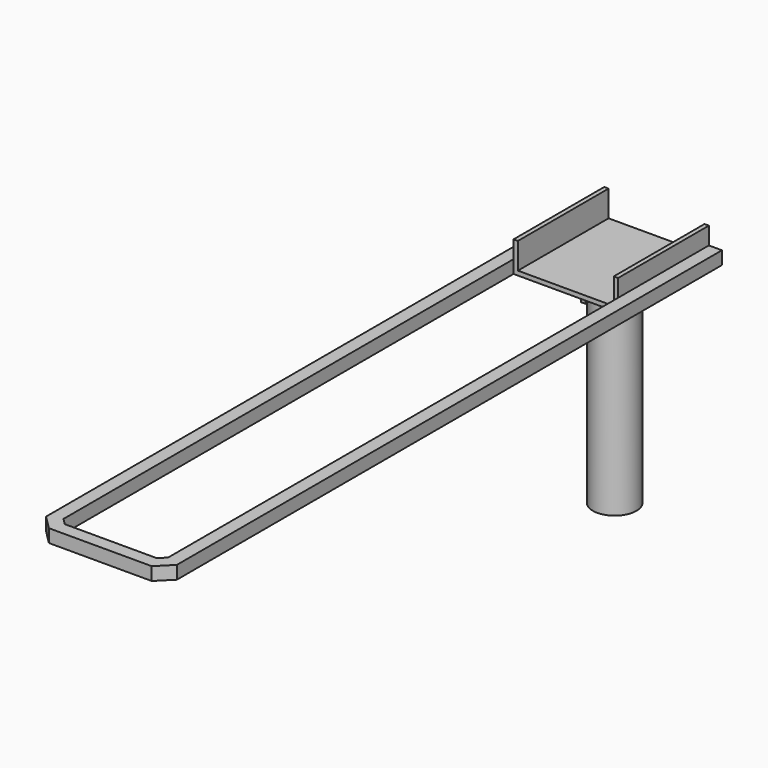
from build123d import *

# Parameters (mm, degrees)
F0_R     = 31.75
F0_R_2   = 28.575
F1_DEPTH = 304.8
F2_W     = 6.35
F2_H     = 28.575
F3_DEPTH = 25.4
F6_DEPTH = 165.1
F7_W     = 19.05
F7_H     = 19.05
F7_W_2   = 12.7
F7_H_2   = 12.7


# Not quite as in the source:
# - a feature names something its author has since deleted; it is built from what else it names


with BuildPart() as f1:
    # F0 (on Top) → F1 (new body)
    with BuildSketch(Plane.XY):
        Circle(F0_R)
        Circle(F0_R_2, mode=Mode.SUBTRACT)
    extrude(amount=-F1_DEPTH)

    # F2 (on Top) → F3 (join)
    with BuildSketch(Plane.XY):
        with Locations((0, -42.8625)):
            Rectangle(F2_W, F2_H)
    extrude(amount=-F3_DEPTH)

    # F5 (on offset) → F6 (join)
    with BuildSketch(Plane.XZ.offset(-76.2)):
        Polygon((-76.2, 0), (76.2, 0), (76.2, 44.45), (69.85, 44.45), (69.85, 6.35), (-69.85, 6.35), (-69.85, 44.45), (-76.2, 44.45), align=None)
    extrude(amount=F6_DEPTH)

    # F9: sweep along a path in F8
    with BuildLine(Plane.XY.offset(6.35)) as f9_path:
        Line((98.425, 76.2), (98.425, -917.575))
        Line((98.425, -917.575), (76.2, -939.8))
        Line((76.2, -939.8), (-76.2, -939.8))
        Line((-76.2, -939.8), (-98.425, -917.575))
        Line((-98.425, -917.575), (-98.425, 76.2))
    # F7 (on offset) → F9 (sweep)
    with BuildSketch(Plane.XZ.offset(-76.2)):
        with Locations((85.725, 9.525)):
            Rectangle(F7_W, F7_H)
        with Locations((85.725, 9.525)):
            Rectangle(F7_W_2, F7_H_2, mode=Mode.SUBTRACT)
    sweep(path=f9_path.line, transition=Transition.RIGHT)


solid = f1.part
